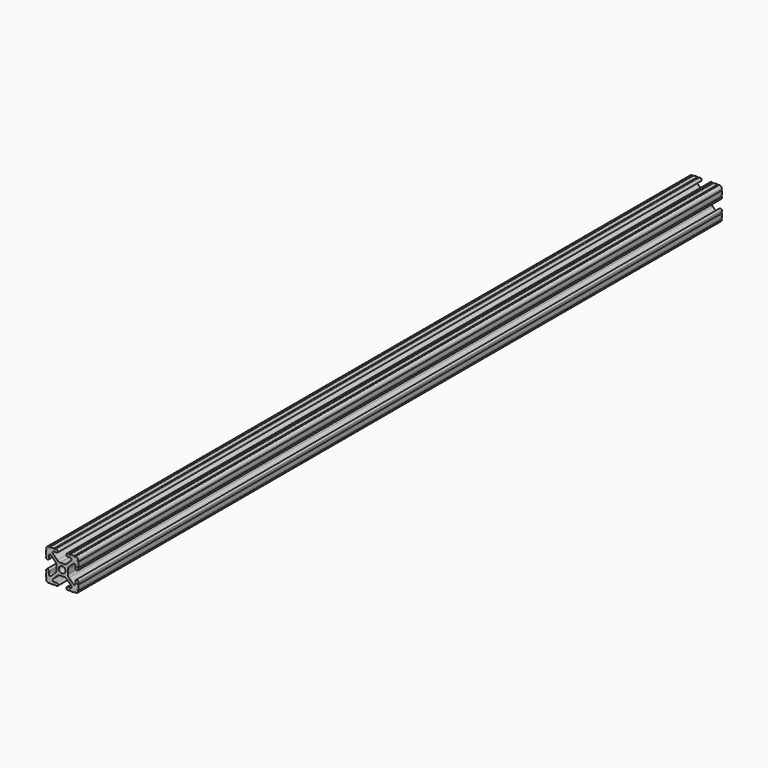
from build123d import *

# Parameters (mm, degrees)
F0_R     = 2.6035
F1_DEPTH = 317.5


# Not quite as in the source:
# - ends of sketch curves that miss each other by under 0.0002 mm in the source are joined


with BuildPart() as f1:
    # F0 (on Front) → F1 (new body, symmetric)
    with BuildSketch(Plane.XZ):
        with BuildLine():
            ThreePointArc((-120.045226, 66.1162), (-119.5372260057, 65.6082762), (-120.0450736, 65.1002000229))
            ThreePointArc((-120.0450736, 65.1002000229), (-119.4277485161, 63.5840774839), (-117.9116260074, 62.9667530175))
            ThreePointArc((-117.9116260074, 62.9667530175), (-117.4035498, 63.4745999943), (-116.895626, 62.9666))
            Line((-116.895626, 62.9666), (-113.6783096, 62.9666))
            ThreePointArc((-113.6783096, 62.9666), (-113.1703096, 63.4746), (-112.6623096, 62.9666))
            Line((-112.6623096, 62.9666), (-111.688626, 62.9666))
            ThreePointArc((-111.688626, 62.9666), (-110.583726, 64.0715), (-111.688626, 65.1764))
            Line((-111.688626, 65.1764), (-113.8200162, 65.1764))
            ThreePointArc((-113.8200162, 65.1764), (-114.758677805, 65.8035936327), (-114.5384366897, 66.9108204897))
            Line((-114.5384366897, 66.9108204897), (-111.2083882, 70.2408552))
            ThreePointArc((-111.2083882, 70.2408552), (-110.1783528978, 70.9291175157), (-108.963333, 71.1708))
            Line((-108.963333, 71.1708), (-105.727119, 71.1708))
            ThreePointArc((-105.727119, 71.1708), (-104.5120991022, 70.9291175157), (-103.4820549697, 70.2408640303))
            Line((-103.4820549697, 70.2408640303), (-100.1520222, 66.9108136))
            ThreePointArc((-100.1520222, 66.9108136), (-99.931774195, 65.8035936327), (-100.8704358, 65.1764))
            Line((-100.8704358, 65.1764), (-103.001826, 65.1764))
            ThreePointArc((-103.001826, 65.1764), (-104.106726, 64.0715), (-103.001826, 62.9666))
            Line((-103.001826, 62.9666), (-102.0281424, 62.9666))
            ThreePointArc((-102.0281424, 62.9666), (-101.5201424, 63.4746), (-101.0121424, 62.9666))
            Line((-101.0121424, 62.9666), (-97.794826, 62.9666))
            ThreePointArc((-97.794826, 62.9666), (-97.2869022, 63.4745999943), (-96.7788260229, 62.9667524))
            ThreePointArc((-96.7788260229, 62.9667524), (-95.2627034839, 63.5840774839), (-94.6453790175, 65.1001999926))
            ThreePointArc((-94.6453790175, 65.1001999926), (-95.1532259943, 65.6082762), (-94.645226, 66.1162))
            Line((-94.645226, 66.1162), (-94.645226, 69.3335164))
            ThreePointArc((-94.645226, 69.3335164), (-95.153226, 69.8415164), (-94.645226, 70.3495164))
            Line((-94.645226, 70.3495164), (-94.645226, 71.3232))
            ThreePointArc((-94.645226, 71.3232), (-95.750126, 72.4281), (-96.855026, 71.3232))
            Line((-96.855026, 71.3232), (-96.855026, 69.1918098))
            ThreePointArc((-96.855026, 69.1918098), (-97.4822196327, 68.253148195), (-98.5894464897, 68.4733893103))
            Line((-98.5894464897, 68.4733893103), (-101.9194812, 71.8034378))
            ThreePointArc((-101.9194812, 71.8034378), (-102.6077435157, 72.8334731022), (-102.849426, 74.048493))
            Line((-102.849426, 74.048493), (-102.849426, 77.284707))
            ThreePointArc((-102.849426, 77.284707), (-102.6077435157, 78.4997268978), (-101.9194900303, 79.5297710303))
            Line((-101.9194900303, 79.5297710303), (-98.5894396, 82.8598038))
            ThreePointArc((-98.5894396, 82.8598038), (-97.4822196327, 83.080051805), (-96.855026, 82.1413902))
            Line((-96.855026, 82.1413902), (-96.855026, 80.01))
            ThreePointArc((-96.855026, 80.01), (-95.750126, 78.9051), (-94.645226, 80.01))
            Line((-94.645226, 80.01), (-94.645226, 80.9836836))
            ThreePointArc((-94.645226, 80.9836836), (-95.153226, 81.4916836), (-94.645226, 81.9996836))
            Line((-94.645226, 81.9996836), (-94.645226, 85.217))
            ThreePointArc((-94.645226, 85.217), (-95.1532259943, 85.7249238), (-94.6453784, 86.2329999771))
            ThreePointArc((-94.6453784, 86.2329999771), (-95.2627034839, 87.7491225161), (-96.7788259926, 88.3664469825))
            ThreePointArc((-96.7788259926, 88.3664469825), (-97.2869022, 87.8586000057), (-97.794826, 88.3666))
            Line((-97.794826, 88.3666), (-101.0121424, 88.3666))
            ThreePointArc((-101.0121424, 88.3666), (-101.5201424, 87.8586), (-102.0281424, 88.3666))
            Line((-102.0281424, 88.3666), (-103.001826, 88.3666))
            ThreePointArc((-103.001826, 88.3666), (-104.106726, 87.2617), (-103.001826, 86.1568))
            Line((-103.001826, 86.1568), (-100.8704358, 86.1568))
            ThreePointArc((-100.8704358, 86.1568), (-99.931774195, 85.5296063673), (-100.1520153103, 84.4223795103))
            Line((-100.1520153103, 84.4223795103), (-103.4820638, 81.0923448))
            ThreePointArc((-103.4820638, 81.0923448), (-104.5120991022, 80.4040824843), (-105.727119, 80.1624))
            Line((-105.727119, 80.1624), (-108.963333, 80.1624))
            ThreePointArc((-108.963333, 80.1624), (-110.1783528978, 80.4040824843), (-111.2083970303, 81.0923359697))
            Line((-111.2083970303, 81.0923359697), (-114.5384298, 84.4223864))
            ThreePointArc((-114.5384298, 84.4223864), (-114.758677805, 85.5296063673), (-113.8200162, 86.1568))
            Line((-113.8200162, 86.1568), (-111.688626, 86.1568))
            ThreePointArc((-111.688626, 86.1568), (-110.583726, 87.2617), (-111.688626, 88.3666))
            Line((-111.688626, 88.3666), (-112.6623096, 88.3666))
            ThreePointArc((-112.6623096, 88.3666), (-113.1703096, 87.8586), (-113.6783096, 88.3666))
            Line((-113.6783096, 88.3666), (-116.895626, 88.3666))
            ThreePointArc((-116.895626, 88.3666), (-117.4035498, 87.8586000057), (-117.9116259771, 88.3664476))
            ThreePointArc((-117.9116259771, 88.3664476), (-119.4277485161, 87.7491225161), (-120.0450729825, 86.2330000074))
            ThreePointArc((-120.0450729825, 86.2330000074), (-119.5372260057, 85.7249238), (-120.045226, 85.217))
            Line((-120.045226, 85.217), (-120.045226, 81.9996836))
            ThreePointArc((-120.045226, 81.9996836), (-119.537226, 81.4916836), (-120.045226, 80.9836836))
            Line((-120.045226, 80.9836836), (-120.045226, 80.01))
            ThreePointArc((-120.045226, 80.01), (-118.940326, 78.9051), (-117.835426, 80.01))
            Line((-117.835426, 80.01), (-117.835426, 82.1413902))
            ThreePointArc((-117.835426, 82.1413902), (-117.2082323673, 83.080051805), (-116.1010055103, 82.8598106897))
            Line((-116.1010055103, 82.8598106897), (-112.7709708, 79.5297622))
            ThreePointArc((-112.7709708, 79.5297622), (-112.0827084843, 78.4997268978), (-111.841026, 77.284707))
            Line((-111.841026, 77.284707), (-111.841026, 74.048493))
            ThreePointArc((-111.841026, 74.048493), (-112.0827084843, 72.8334731022), (-112.7709619697, 71.8034289697))
            Line((-112.7709619697, 71.8034289697), (-116.1010124, 68.4733962))
            ThreePointArc((-116.1010124, 68.4733962), (-117.2082323673, 68.253148195), (-117.835426, 69.1918098))
            Line((-117.835426, 69.1918098), (-117.835426, 71.3232))
            ThreePointArc((-117.835426, 71.3232), (-118.940326, 72.4281), (-120.045226, 71.3232))
            Line((-120.045226, 71.3232), (-120.045226, 70.3495164))
            ThreePointArc((-120.045226, 70.3495164), (-119.537226, 69.8415164), (-120.045226, 69.3335164))
            Line((-120.045226, 69.3335164), (-120.045226, 66.1162))
        make_face()
        with Locations((-107.345226, 75.6666)):
            Circle(F0_R, mode=Mode.SUBTRACT)
    extrude(amount=F1_DEPTH, both=True)


solid = f1.part
